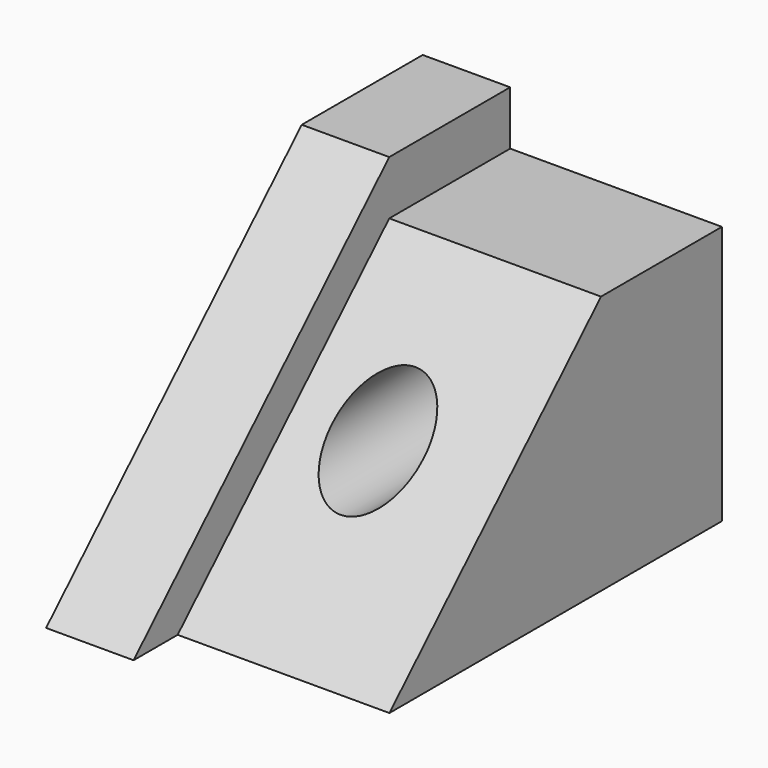
from build123d import *

# Parameters (mm, degrees)
F1_DEPTH = 30.734
F2_DEPTH = 12.7
F3_R     = 6.6708512145
F4_DEPTH = 45.212
F5_DEPTH = 29.972


# Not quite as in the source:
# - a feature names something its author has since deleted; it is built from what else it names


with BuildPart() as f1:
    # F0 (on Right) → F1 (new body)
    with BuildSketch(Plane.YZ):
        Polygon((-28.4980535507, 0), (31.8277217448, 0), (31.8277217448, 37.6056805253), (9.8910769448, 37.6056805253), align=None)
    extrude(amount=F1_DEPTH)

    # F0 (on Right) → F2 (join)
    with BuildSketch(Plane.YZ):
        Polygon((-28.4980535507, 0), (31.8277217448, 0), (31.8277217448, 37.6056805253), (9.8910769448, 37.6056805253), align=None)
        Polygon((9.8910769448, 37.6056805253), (31.8277217448, 37.6056805253), (31.8277217448, 45.440196991), (9.8910769448, 45.440196991), (-36.4957887537, 0), (-28.4980535507, 0), align=None)
    extrude(amount=-F2_DEPTH)

    # F3 (on Front) → F4 (cut)
    with BuildSketch(Plane.XZ):
        with Locations((12.4372942373, 20.3697439283)):
            Circle(F3_R)
    extrude(amount=-F4_DEPTH, mode=Mode.SUBTRACT)

    # F3 (on Front) → F5 (cut)
    with BuildSketch(Plane.XZ):
        with Locations((12.4372942373, 20.3697439283)):
            Circle(F3_R)
    extrude(amount=F5_DEPTH, mode=Mode.SUBTRACT)


solid = f1.part
